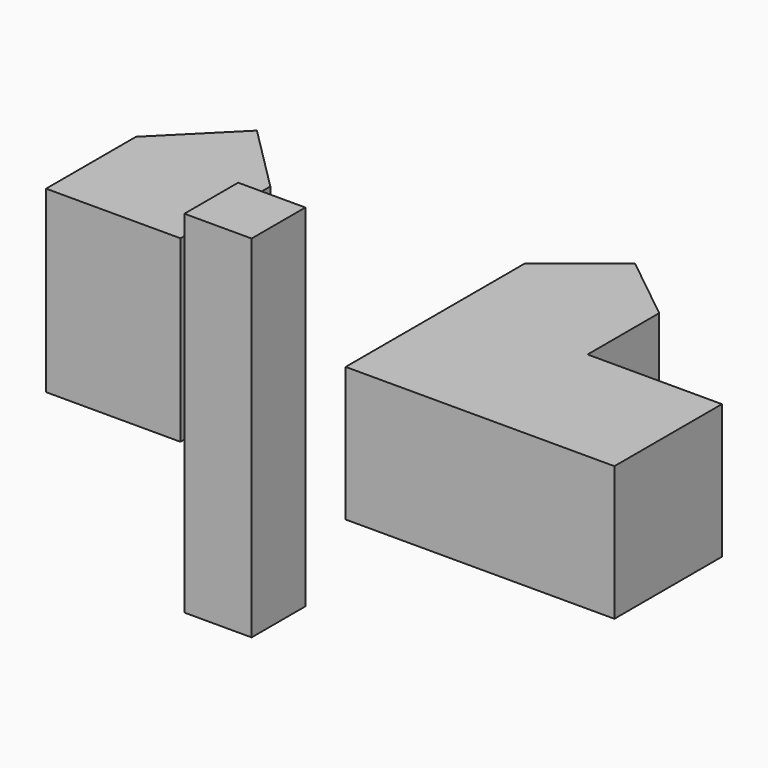
from build123d import *

# Parameters (mm, degrees)
F1_DEPTH = 9.525
F3_DEPTH = 12.7
F4_W     = 4.7625
F4_H     = 4.7625
F5_DEPTH = 24.892


# Not quite as in the source:
# - a length typed as a fraction of an inch, garbled in the dataset ("3 / 203.2 mm" for 3/8 in), is restored


with BuildPart() as f1:
    # F0 (on Top) → F1 (new body)
    with BuildSketch(Plane.XY):
        Polygon((19.05, -9.525), (19.05, 0), (9.525, 0), (9.525, 6.35), (4.7625, 10.16), (0, 6.35), (0, 0), (0, -9.525), align=None)
    extrude(amount=F1_DEPTH)


with BuildPart() as f3:
    # F2 (on Top) → F3 (new body)
    with BuildSketch(Plane.XY):
        Polygon((-22.4840769566, 0), (-22.4840769566, -7.9629), (-12.9590769566, -7.9629), (-12.9590769566, 0), (-17.7215769566, 4.7625), align=None)
    extrude(amount=F3_DEPTH)


with BuildPart() as f5:
    # F4 (on Top) → F5 (new body)
    with BuildSketch(Plane.XY):
        with Locations((2.38125, -21.43125)):
            Rectangle(F4_W, F4_H)
    extrude(amount=F5_DEPTH)


solid = Compound([f1.part, f3.part, f5.part])
